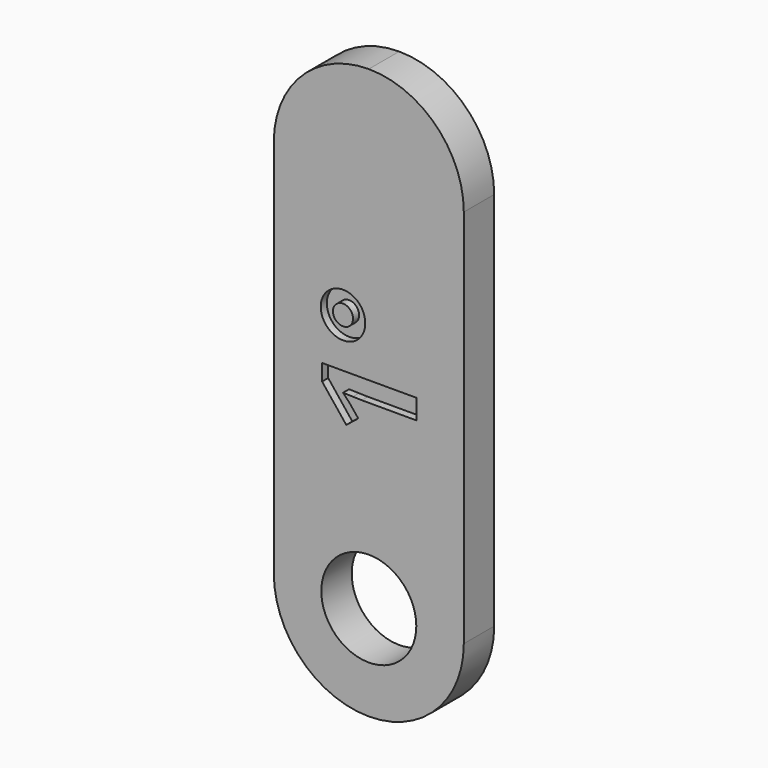
from build123d import *

# Parameters (mm, degrees)
F0_W         = 12.7
F0_H         = 38.1
F0_R         = 3.175
F1_DEPTH     = 2.54
F2_R         = 6.34999
F3_TEXT_SIZE = 8.8194444444
F4_DEPTH     = 0.508


# Not quite as in the source:
# - a fillet or chamfer is up to 0.001 mm smaller than in the source, because OpenCascade refuses the exact size
# - Text() gives the source's letters only with a copy of the font that has no kerning and outlines rounded to 1/6400 em; it was checked with that copy


with BuildPart() as f1:
    # F0 (on Front) → F1 (new body)
    with BuildSketch(Plane.XZ):
        with Locations((6.35, 19.05)):
            Rectangle(F0_W, F0_H)
        with Locations((6.35, 6.35)):
            Circle(F0_R, mode=Mode.SUBTRACT)
    extrude(amount=F1_DEPTH)

    # F2 (radius 6.35 in the source; OpenCascade refuses exactly that, so slightly less here)
    f2_edges = [f1.edges().sort_by_distance(p)[0] for p in [
        (12.7, -1.27, 0),
        (0, -1.27, 0),
        (12.7, -1.27, 38.1),
        (0, -1.27, 38.1),
    ]]
    fillet(f2_edges, radius=F2_R)

    # F3 (on face) → F4 (cut)
    with BuildSketch(Plane.XZ.offset(2.54)):
        with Locations(Location((9.525, 16.1464735243), (0, 0, 90))):
            Text('1°', F3_TEXT_SIZE, font='Open Sans', font_style=FontStyle.BOLD, text_align=(TextAlign.LEFT, TextAlign.BOTTOM))
    extrude(amount=-F4_DEPTH, mode=Mode.SUBTRACT)


solid = f1.part
